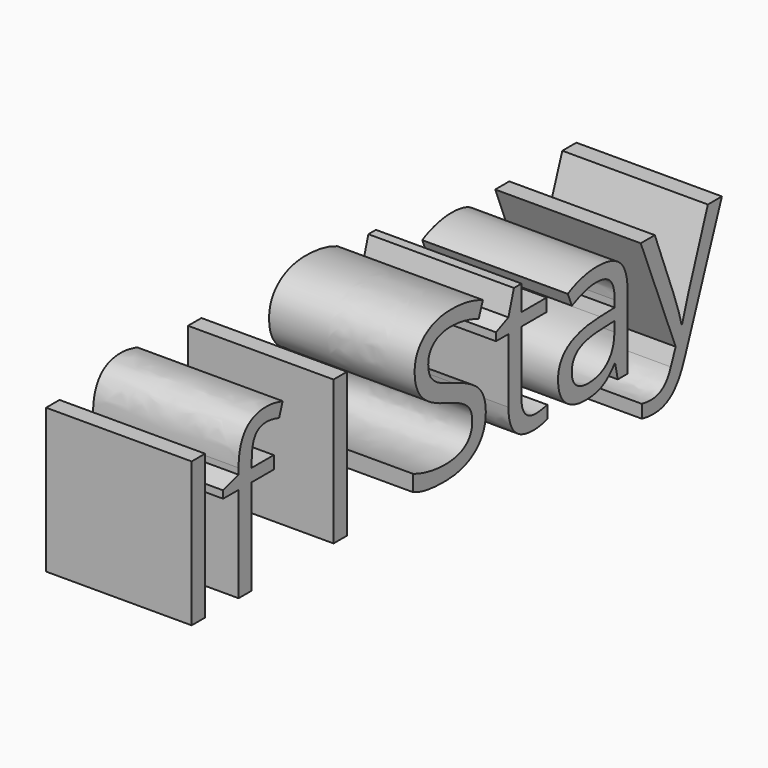
from build123d import *

# Parameters (mm, degrees)
F0_TEXT_SIZE = 17.6388888889
F1_DEPTH     = 12.7


# Not quite as in the source:
# - Text() gives the source's letters only with a copy of the font that has no kerning and outlines rounded to 1/6400 em; it was checked with that copy


with BuildPart() as f1:
    # F0 (on Right) → F1 (new body)
    with BuildSketch(Plane.YZ):
        with Locations((-41.8522874732, 25.2075855882)):
            Text('If I Stay', F0_TEXT_SIZE, font='Open Sans', text_align=(TextAlign.LEFT, TextAlign.BOTTOM))
    extrude(amount=F1_DEPTH)


solid = f1.part
